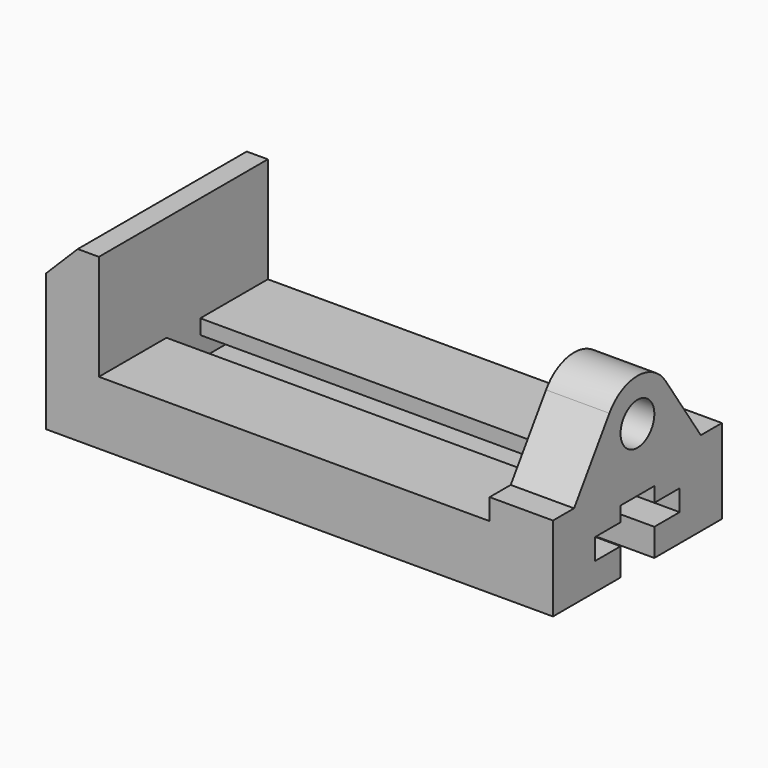
from build123d import *

# Parameters (mm, degrees)
F1_DEPTH = 4.625
F2_R     = 0.5
F3_DEPTH = 1.5
F5_DEPTH = 1.25
F6_SIZE2 = 0.75
F6_SIZE  = 0.75


with BuildPart() as f1:
    # F0 (on Right) → F1 (new body, symmetric)
    with BuildSketch(Plane.YZ):
        Polygon((0, 1.5), (0, 0), (2, 0), (2, 0.65), (1.25, 0.65), (1.25, 1.15), (2, 1.15), (2, 1.5), align=None)
    extrude(amount=F1_DEPTH, both=True)



with BuildPart() as f1b:
    # F0 (on Right) → F1, piece 2 (new body, symmetric)
    with BuildSketch(Plane.YZ):
        Polygon((3, 0.65), (3, 0), (5, 0), (5, 1.5), (3, 1.5), (3, 1.15), (3.75, 1.15), (3.75, 0.65), align=None)
    extrude(amount=F1_DEPTH, both=True)


with BuildPart() as f1_1:
    add(f1.part)

    add(f1b.part)  # F3 merges F1b
    # F2 (on face) → F3 (join)
    with BuildSketch(Plane.YZ.offset(4.625)):
        with BuildLine():
            Line((0, 2), (0, 1.5))
            Line((0, 1.5), (2, 1.5))
            Line((2, 1.5), (3, 1.5))
            Line((3, 1.5), (3, 1.15))
            Line((3, 1.15), (3.75, 1.15))
            Line((3.75, 1.15), (3.75, 0.65))
            Line((3.75, 0.65), (3, 0.65))
            Line((3, 0.65), (3, 0))
            Line((3, 0), (5, 0))
            Line((5, 0), (5, 2))
            Line((5, 2), (4.375, 2))
            Line((4.375, 2), (3.330449827, 3.5570934256))
            ThreePointArc((3.330449827, 3.5570934256), (2.5, 4), (1.669550173, 3.5570934256))
            Line((1.669550173, 3.5570934256), (0.625, 2))
            Line((0.625, 2), (0, 2))
        make_face()
        with Locations((2.5, 3)):
            Circle(F2_R, mode=Mode.SUBTRACT)
        Polygon((0, 1.5), (0, 0), (2, 0), (2, 0.65), (1.25, 0.65), (1.25, 1.15), (2, 1.15), (2, 1.5), align=None)
    extrude(amount=F3_DEPTH)

    # F4 (on face) → F5 (join)
    with BuildSketch(Plane(origin=(-4.625, 0, 0), x_dir=(0, -1, 0), z_dir=(-1, 0, 0))):
        Polygon((-5, 1.5), (-5, 0), (0, 0), (0, 4), (-5, 4), align=None)
    extrude(amount=F5_DEPTH)

    # F6
    f6_edges = [f1_1.edges().sort_by_distance(p)[0] for p in [
        (-5.875, 2.5, 4),
    ]]
    chamfer(f6_edges, length=F6_SIZE, length2=F6_SIZE2)


solid = f1_1.part
